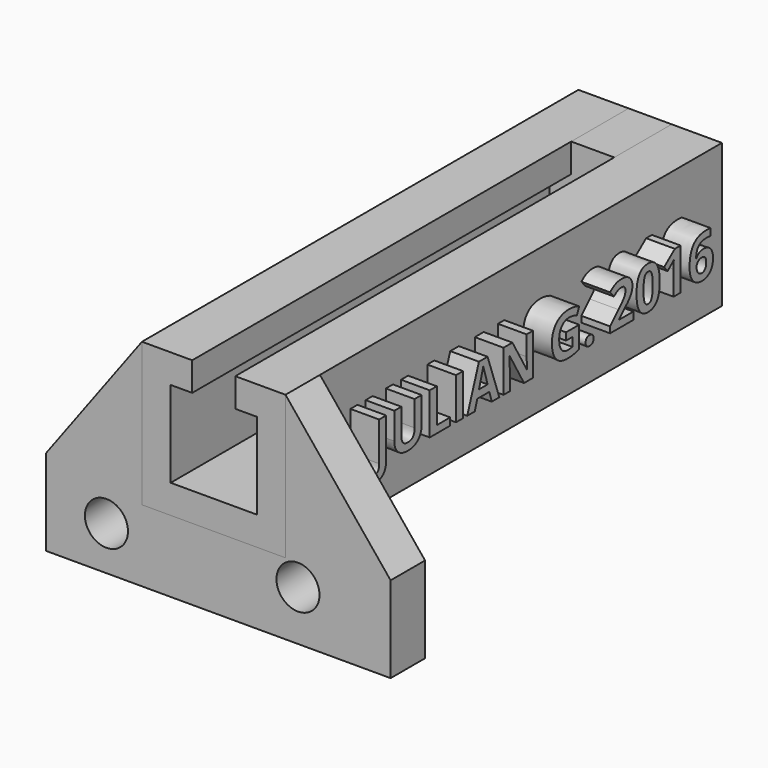
from build123d import *

# Parameters (mm, degrees)
F1_DEPTH     = 38
F0_R         = 1.5
F2_DEPTH     = 3
F0_W         = 3
F0_H         = 2
F3_DEPTH     = 38
F4_DEPTH     = 33
F5_TEXT_SIZE = 4.0510602384
F6_DEPTH     = 2


# Not quite as in the source:
# - Text() gives the source's letters only with a copy of the font that has no kerning and outlines rounded to 1/6400 em; it was checked with that copy


with BuildPart() as f1:
    # F0 (on Front) → F1 (new body)
    with BuildSketch(Plane.XZ):
        Polygon((10.1783145999, 0), (6.6783145999, 0), (6.6783145999, -10), (16.6783145999, -10), (16.6783145999, 0), (13.1783145999, 0), (13.1783145999, -2), (14.6783145999, -2), (14.6783145999, -8), (8.6783145999, -8), (8.6783145999, -2), (10.1783145999, -2), align=None)
    extrude(amount=-F1_DEPTH)

    # F5 (on face) → F6 (join)
    with BuildSketch(Plane.YZ.offset(16.6783145999)):
        with Locations((5.288935027, -6.0577187015)):
            Text('JULIAN G. 2016', F5_TEXT_SIZE, font='Open Sans', font_style=FontStyle.BOLD, text_align=(TextAlign.LEFT, TextAlign.BOTTOM))
    extrude(amount=F6_DEPTH)


with BuildPart() as f2:
    # F0 (on Front) → F2 (new body)
    with BuildSketch(Plane.XZ):
        Polygon((6.6783145999, -10), (6.6783145999, 0), (0, -9), (0, -15), (24, -15), (24, -9), (16.6783145999, 0), (16.6783145999, -10), align=None)
        with Locations((4.2050299235, -11.9438655674)):
            Circle(F0_R, mode=Mode.SUBTRACT)
        with Locations((17.5476651639, -11.513219215)):
            Circle(F0_R, mode=Mode.SUBTRACT)
    extrude(amount=-F2_DEPTH)


with BuildPart() as f3:
    # F0 (on Front) → F3 (new body)
    with BuildSketch(Plane.XZ):
        Polygon((13.1783145999, -2), (10.1783145999, -2), (8.6783145999, -2), (8.6783145999, -8), (14.6783145999, -8), (14.6783145999, -2), align=None)
        with Locations((11.6783145999, -1)):
            Rectangle(F0_W, F0_H)
    extrude(amount=-F3_DEPTH)

    # F0 (on Front) → F4 (cut)
    with BuildSketch(Plane.XZ):
        Polygon((13.1783145999, -2), (10.1783145999, -2), (8.6783145999, -2), (8.6783145999, -8), (14.6783145999, -8), (14.6783145999, -2), align=None)
        with Locations((11.6783145999, -1)):
            Rectangle(F0_W, F0_H)
    extrude(amount=-F4_DEPTH, mode=Mode.SUBTRACT)


solid = Compound([f1.part, f2.part, f3.part])
